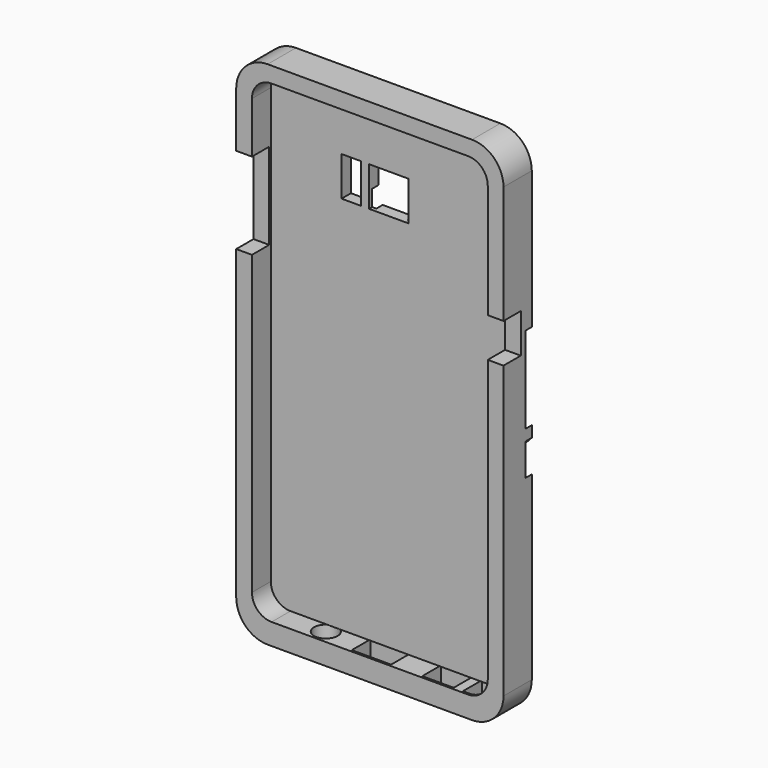
from build123d import *

# Parameters (mm, degrees)
F1_DEPTH     = 8.89
F3_DEPTH     = 7.62
F5_R         = 3.81
F6_DEPTH     = 6.858
F8_T1_DEPTH  = 7.62
F8_T6_DEPTH  = 7.62
F8_T12_DEPTH = 7.62
F8_T18_DEPTH = 7.62
F10_DEPTH    = 25.4
F12_DEPTH    = 25.4
F13_W        = 6.35
F13_H        = 12.7
F14_DEPTH    = 25.4
F15_DEPTH    = 2.54
F16_T1_DEPTH = 62.23
F17_DEPTH    = 2.54
F19_DEPTH    = 11.431
F20_W        = 2.5078685576
F20_H        = 12.7
F21_DEPTH    = 12.7
F23_DEPTH    = 12.7
F25_DEPTH    = 12.7


# Not quite as in the source:
# - a fillet or chamfer that OpenCascade refuses, or shapes differently, is made with other operations: its cross-section is extruded or revolved along the edge and cut away or added
# - a feature of the source that left no trace in its solid (it failed there, or was rolled back) is left out


with BuildPart() as f1:
    # F0 (on Front) → F1 (new body)
    with BuildSketch(Plane.XZ):
        Polygon((0, 82.55), (0, 0), (0, -82.55), (43.18, -82.55), (43.18, 82.55), align=None)
        Polygon((0, -82.55), (0, 0), (0, 82.55), (-43.18, 82.55), (-43.18, -82.55), align=None)
    extrude(amount=F1_DEPTH)

    # F2 (on face) → F3 (cut)
    with BuildSketch(Plane.XZ.offset(8.89)):
        Polygon((38.1, 77.47), (0, 77.47), (-38.1, 77.47), (-38.1, -75.692), (38.1, -75.692), align=None)
    extrude(amount=-F3_DEPTH, mode=Mode.SUBTRACT)

    # F5 (on face) → F6 (cut)
    with BuildSketch(Plane(origin=(0, 0, -82.55), x_dir=(1, 0, 0), z_dir=(0, 0, -1))):
        with Locations((-17.78, 4.445)):
            Circle(F5_R)
        Polygon((6.35, 0.635), (6.35, 4.445), (6.35, 8.255), (-6.35, 8.255), (-6.35, 0.635), align=None)
        Polygon((16.4221003652, 8.255), (16.4221003652, 4.445), (16.4221003652, 0.635), (26.5821003652, 0.635), (26.5821003652, 8.255), align=None)
        Polygon((29.568027705, 8.255), (29.568027705, 4.445), (29.568027705, 0.635), (37.188027705, 0.635), (37.188027705, 8.255), align=None)
    extrude(amount=-F6_DEPTH, mode=Mode.SUBTRACT)

    # F8: fillet of radius 6.35 on 4 edges, made by hand

    # F8_s2 → F8_t1 (join)
    with BuildSketch(Plane.XZ.offset(1.27)):
        with BuildLine():
            ThreePointArc((-38.1, -69.342), (-36.2401280605, -73.8321280605), (-31.75, -75.692))
            Line((-31.75, -75.692), (-38.1, -75.692))
            Line((-38.1, -75.692), (-38.1, -69.342))
        make_face()
        with BuildLine():
            ThreePointArc((-38.1, 71.12), (-36.2401280605, 75.6101280605), (-31.75, 77.47))
            Line((-31.75, 77.47), (-38.1, 77.47))
            Line((-38.1, 77.47), (-38.1, 71.12))
        make_face()
        with BuildLine():
            ThreePointArc((38.1, 71.12), (36.2401280605, 75.6101280605), (31.75, 77.47))
            Line((31.75, 77.47), (38.1, 77.47))
            Line((38.1, 77.47), (38.1, 71.12))
        make_face()
    extrude(amount=F8_T1_DEPTH)


with BuildPart() as f8_tool4:
    # F8_s5 → F8_t6 (new body)
    with BuildSketch(Plane.XZ.offset(8.89)):
        with BuildLine():
            ThreePointArc((31.75, -75.692), (36.2401280605, -73.8321280605), (38.1, -69.342))
            Line((38.1, -69.342), (38.1, -75.692))
            Line((38.1, -75.692), (31.75, -75.692))
        make_face()
    extrude(amount=-F8_T6_DEPTH)

    split(bisect_by=Plane.YZ.offset(37.188027705), keep=Keep.BOTTOM)

    split(bisect_by=Plane.XZ.offset(8.255), keep=Keep.TOP)


with BuildPart() as f1_1:
    add(f1.part)

    # F8_t3: union F8_tool4
    add(f8_tool4.part)


with BuildPart() as f8_tool10:
    # F8_s11 → F8_t12 (new body)
    with BuildSketch(Plane.XZ.offset(8.89)):
        with BuildLine():
            ThreePointArc((31.75, -75.692), (36.2401280605, -73.8321280605), (38.1, -69.342))
            Line((38.1, -69.342), (38.1, -75.692))
            Line((38.1, -75.692), (31.75, -75.692))
        make_face()
    extrude(amount=-F8_T12_DEPTH)

    split(bisect_by=Plane.YZ.offset(37.188027705), keep=Keep.TOP)

    split(bisect_by=Plane.XZ.offset(8.255), keep=Keep.TOP)


with BuildPart() as f1_2:
    add(f1_1.part)

    # F8_t9: union F8_tool10
    add(f8_tool10.part)


with BuildPart() as f8_tool16:
    # F8_s17 → F8_t18 (new body)
    with BuildSketch(Plane.XZ.offset(8.89)):
        with BuildLine():
            ThreePointArc((31.75, -75.692), (36.2401280605, -73.8321280605), (38.1, -69.342))
            Line((38.1, -69.342), (38.1, -75.692))
            Line((38.1, -75.692), (31.75, -75.692))
        make_face()
    extrude(amount=-F8_T18_DEPTH)

    split(bisect_by=Plane.YZ.offset(37.188027705), keep=Keep.TOP)

    split(bisect_by=Plane.XZ.offset(8.255), keep=Keep.BOTTOM)


with BuildPart() as f1_3:
    add(f1_2.part)

    # F8_t15: union F8_tool16
    add(f8_tool16.part)

    # F9 (on face) → F10 (cut)
    with BuildSketch(Plane.YZ.offset(43.18)):
        Polygon((-6.985, 21.59), (-4.445, 21.59), (-1.905, 21.59), (-1.905, 34.29), (-6.985, 34.29), align=None)
    extrude(amount=-F10_DEPTH, mode=Mode.SUBTRACT)

    # F11 (on face) → F12 (cut)
    with BuildSketch(Plane(origin=(-43.18, 0, 0), x_dir=(0, -1, 0), z_dir=(-1, 0, 0))):
        Polygon((1.905, 26.67), (4.445, 26.67), (6.985, 26.67), (6.985, 39.37), (1.905, 39.37), align=None)
        Polygon((1.905, 41.91), (4.445, 41.91), (6.985, 41.91), (6.985, 54.61), (1.905, 54.61), align=None)
    extrude(amount=-F12_DEPTH, mode=Mode.SUBTRACT)

    # F13 (on face) → F14 (cut)
    with BuildSketch(Plane(origin=(0, 0, 0), x_dir=(-1, 0, 0), z_dir=(0, 1, 0))):
        with Locations((3.175, 53.34)):
            Rectangle(F13_W, F13_H)
        with Locations((-3.175, 53.34)):
            Rectangle(F13_W, F13_H)
        with Locations((12.065, 53.34)):
            Rectangle(F13_W, F13_H)
    extrude(amount=-F14_DEPTH, mode=Mode.SUBTRACT)

    # F4 (on face) → F15 (join)
    with BuildSketch(Plane(origin=(0, 0, 0), x_dir=(-1, 0, 0), z_dir=(0, 1, 0))):
        with BuildLine():
            Line((-43.18, 82.55), (-43.18, 27.94))
            add(Edge.make_bspline(
                [(-43.18, 27.94), (-34.3400128186, 42.8215824068), (-27.4204702229, 48.0896333512), (-16.0427556486, 49.7445749399)],
                knots=[0, 0, 0, 0, 34.8119163405, 34.8119163405, 34.8119163405, 34.8119163405], degree=3))
            add(Edge.make_bspline(
                [(-16.0427556486, 49.7445749399), (-21.9130860807, 37.157849131), (-27.3593299999, 28.3380299427), (-10.0758119389, 22.9448514021), (-9.5159057528, 43.6490513384), (-8.3359745983, 54.9122218837)],
                knots=[0, 0, 0, 0, 0.3657981672, 0.5856406882, 1, 1, 1, 1], degree=3))
            add(Edge.make_bspline(
                [(-8.3359745983, 54.9122218837), (-6.046301593, 54.4916797927), (-5.5332067241, 47.6679994945), (-4.1373502463, 44.0627858043)],
                knots=[0, 0, 0, 0, 11.6335166519, 11.6335166519, 11.6335166519, 11.6335166519], degree=3))
            ThreePointArc((-4.1373502463, 44.0627858043), (-2.0978831027, 44.5995830025), (0, 44.8151379824))
            ThreePointArc((0, 44.8151379824), (2.0978831027, 44.5995830025), (4.1373502463, 44.0627858043))
            add(Edge.make_bspline(
                [(8.3359745983, 54.9122218837), (6.046301593, 54.4916797927), (5.5332067241, 47.6679994945), (4.1373502463, 44.0627858043)],
                knots=[0, 0, 0, 0, 11.6335166519, 11.6335166519, 11.6335166519, 11.6335166519], degree=3))
            add(Edge.make_bspline(
                [(16.0427556486, 49.7445749399), (21.9130860807, 37.157849131), (27.3593299999, 28.3380299427), (10.0758119389, 22.9448514021), (9.5159057528, 43.6490513384), (8.3359745983, 54.9122218837)],
                knots=[0, 0, 0, 0, 0.3657981672, 0.5856406882, 1, 1, 1, 1], degree=3))
            add(Edge.make_bspline(
                [(43.18, 27.94), (34.3400128186, 42.8215824068), (27.4204702229, 48.0896333512), (16.0427556486, 49.7445749399)],
                knots=[0, 0, 0, 0, 34.8119163405, 34.8119163405, 34.8119163405, 34.8119163405], degree=3))
            Line((43.18, 27.94), (43.18, 82.55))
            Line((43.18, 82.55), (-43.18, 82.55))
        make_face()
        Polygon((0, -60.6121867895), (-43.18, -13.97), (-43.18, -82.55), (43.18, -82.55), (43.18, -13.97), align=None)
    extrude(amount=F15_DEPTH)

    # F16: fillet of radius 10.16 on 4 edges, made by hand

    # F16_s2 → F16_t1 (cut)
    with BuildSketch(Plane.XZ.offset(-27.94)):
        with BuildLine():
            ThreePointArc((43.18, 72.39), (40.2042048969, 79.5742048969), (33.02, 82.55))
            Line((33.02, 82.55), (43.18, 82.55))
            Line((43.18, 82.55), (43.18, 72.39))
        make_face()
        with BuildLine():
            ThreePointArc((-43.18, 72.39), (-40.2042048969, 79.5742048969), (-33.02, 82.55))
            Line((-33.02, 82.55), (-43.18, 82.55))
            Line((-43.18, 82.55), (-43.18, 72.39))
        make_face()
        with BuildLine():
            ThreePointArc((-43.18, -72.39), (-40.2042048969, -79.5742048969), (-33.02, -82.55))
            Line((-33.02, -82.55), (-43.18, -82.55))
            Line((-43.18, -82.55), (-43.18, -72.39))
        make_face()
        with BuildLine():
            ThreePointArc((43.18, -72.39), (40.2042048969, -79.5742048969), (33.02, -82.55))
            Line((33.02, -82.55), (43.18, -82.55))
            Line((43.18, -82.55), (43.18, -72.39))
        make_face()
    extrude(amount=F16_T1_DEPTH, mode=Mode.SUBTRACT)

    # F4 (on face) → F17 (join)
    with BuildSketch(Plane(origin=(0, 0, 0), x_dir=(-1, 0, 0), z_dir=(0, 1, 0))):
        with BuildLine():
            add(Edge.make_bspline(
                [(-43.18, 0), (-40.1766164425, -2.8449892233), (-36.470121071, -6.3556614495), (-33.6955449991, -4.3492553924), (-33.0948678524, -3.7596412863)],
                knots=[0, 0, 0, 0, 0.0722674677, 0.0926336453, 0.0926336453, 0.0926336453, 0.0926336453], degree=3))
            Line((-43.18, 0), (-43.18, -3.5755655101))
            Line((-43.18, -3.5755655101), (-38.0636267364, -9.1021712869))
            Line((-38.0636267364, -9.1021712869), (-28.2559315046, -19.6962507908))
            ThreePointArc((-28.2559315046, -19.6962507908), (-18.0143879328, -16.3646352707), (-10.8274016529, -24.3856143206))
            ThreePointArc((-10.8274016529, -24.3856143206), (1.5766983654, -27.1611780814), (13.8043301395, -23.6897990108))
            Line((13.8043301395, -23.6897990108), (-33.0948678524, -3.7596412863))
        make_face()
        with BuildLine():
            ThreePointArc((13.8043301395, -35.3065863693), (0, -39.1403292918), (-13.8043301395, -35.3065863693))
            Line((-13.8043301395, -35.3065863693), (0, -50.2177522996))
            Line((0, -50.2177522996), (13.8043301395, -35.3065863693))
        make_face()
        with BuildLine():
            Line((43.18, -3.5755655101), (43.18, 0))
            add(Edge.make_bspline(
                [(-2.525237976, -6.2600033121), (-1.6423205064, -5.6471343085), (0.9763715233, -2.6058289294), (3.4908560435, 0.5668003405), (18.4579647747, 2.1490779239), (9.729226067, -6.1414995128), (17.5111641355, -6.4059065491), (12.9707203551, -13.4560600477), (24.411558477, -5.4708455793), (23.4177332883, 1.5157671495), (32.7497732121, -0.4777995724), (40.2178397356, -0.2382622352), (43.18, 0)],
                knots=[0.4289038826, 0.4289038826, 0.4289038826, 0.4289038826, 0.4589627255, 0.5170602699, 0.5890011946, 0.6440415987, 0.6907809204, 0.7333741401, 0.8038967277, 0.8593314513, 0.9229741114, 1, 1, 1, 1], degree=3))
            Line((-2.525237976, -6.2600033121), (28.4921650697, -19.4410759397))
            Line((28.4921650697, -19.4410759397), (43.18, -3.5755655101))
        make_face()
        with BuildLine():
            add(Edge.make_bspline(
                [(-12.7009608194, -1.9357553524), (-11.5099070026, -0.862057355), (-8.5684333661, 1.6282211357), (-6.9779228581, -2.8853193068), (-5.9654340479, -4.7980667918)],
                knots=[0.3055362492, 0.3055362492, 0.3055362492, 0.3055362492, 0.3382099466, 0.3845833174, 0.3845833174, 0.3845833174, 0.3845833174], degree=3))
            Line((-12.7009608194, -1.9357553524), (-5.9654340479, -4.7980667918))
        make_face()
        with BuildLine():
            add(Edge.make_bspline(
                [(-24.6563881759, 3.1447910766), (-23.0266171617, 3.388297128), (-21.061997043, 2.9227550325), (-19.7710206911, 1.299577146), (-19.5490427282, 0.9743872171)],
                knots=[0.1718970336, 0.1718970336, 0.1718970336, 0.1718970336, 0.2095808225, 0.2181604971, 0.2181604971, 0.2181604971, 0.2181604971], degree=3))
            Line((-24.6563881759, 3.1447910766), (-19.5490427282, 0.9743872171))
        make_face()
    extrude(amount=F17_DEPTH)

    # F18 (on face) → F19 (cut, through all)
    with BuildSketch(Plane(origin=(0, 2.54, 0), x_dir=(-1, 0, 0), z_dir=(0, 1, 0))):
        with BuildLine():
            Line((-5.0040763682, 46.99), (0, 46.99))
            Line((0, 46.99), (5.0040763682, 46.99))
            add(Edge.make_bspline(
                [(6.35, 52.1885766735), (5.8379929325, 50.681298037), (5.4406511405, 48.7628356579), (5.0040763682, 46.99)],
                knots=[4.4190889978, 4.4190889978, 4.4190889978, 4.4190889978, 8.9189348843, 8.9189348843, 8.9189348843, 8.9189348843], degree=3))
            Line((6.35, 52.1885766735), (6.35, 59.69))
            Line((6.35, 59.69), (-6.35, 59.69))
            Line((-6.35, 59.69), (-6.35, 52.1885766735))
            add(Edge.make_bspline(
                [(-6.35, 52.1885766735), (-5.8379929325, 50.681298037), (-5.4406511405, 48.7628356579), (-5.0040763682, 46.99)],
                knots=[4.4190889978, 4.4190889978, 4.4190889978, 4.4190889978, 8.9189348843, 8.9189348843, 8.9189348843, 8.9189348843], degree=3))
        make_face()
        with BuildLine():
            Line((8.89, 59.69), (8.89, 49.0662817784))
            add(Edge.make_bspline(
                [(9.0796624561, 46.99), (9.015448586, 47.680837887), (8.9525937177, 48.3738067628), (8.89, 49.0662817784)],
                knots=[0.9053597033, 0.9053597033, 0.9053597033, 0.9053597033, 0.9299477275, 0.9299477275, 0.9299477275, 0.9299477275], degree=3))
            Line((9.0796624561, 46.99), (15.24, 46.99))
            Line((15.24, 46.99), (15.24, 59.69))
            Line((15.24, 59.69), (8.89, 59.69))
        make_face()
    extrude(amount=-F19_DEPTH, mode=Mode.SUBTRACT)

    # F20 (on face) → F21 (cut)
    with BuildSketch(Plane.YZ.offset(43.18)):
        with Locations((-8.2389342788, 27.94)):
            Rectangle(F20_W, F20_H)
    extrude(amount=-F21_DEPTH, mode=Mode.SUBTRACT)

    # F22 (on face) → F23 (cut)
    with BuildSketch(Plane(origin=(-43.18, 0, 0), x_dir=(0, -1, 0), z_dir=(-1, 0, 0))):
        Polygon((6.985, 41.91), (6.985, 39.37), (6.985, 26.67), (11.1803514883, 26.67), (11.1803514883, 54.61), (6.985, 54.61), align=None)
    extrude(amount=-F23_DEPTH, mode=Mode.SUBTRACT)

    # F24 (on face) → F25 (cut)
    with BuildSketch(Plane(origin=(-43.18, 0, 0), x_dir=(0, -1, 0), z_dir=(-1, 0, 0))):
        Polygon((1.905, 41.91), (1.905, 39.37), (6.985, 39.37), (6.985, 41.91), (4.445, 41.91), align=None)
    extrude(amount=-F25_DEPTH, mode=Mode.SUBTRACT)


solid = f1_3.part
